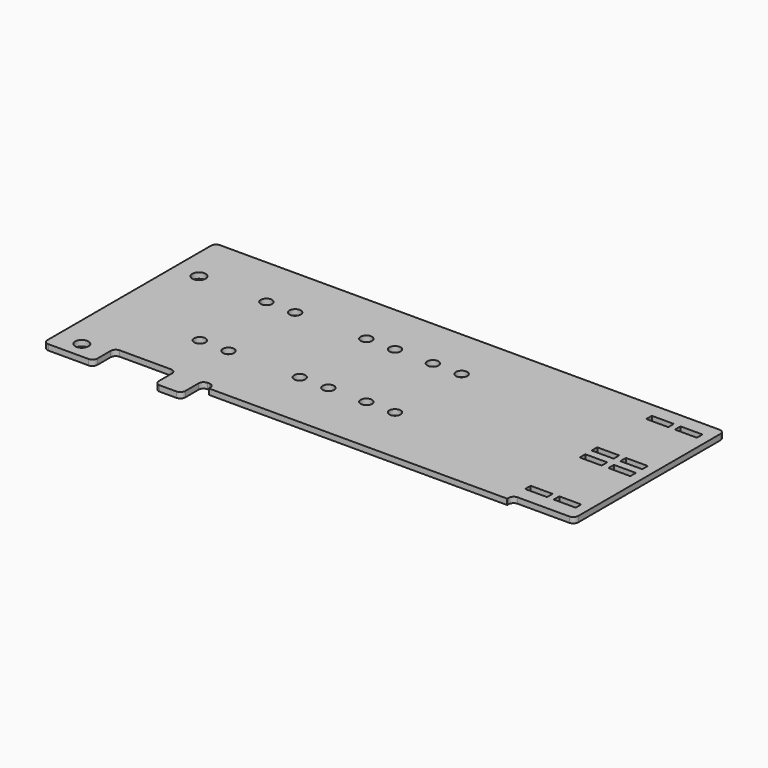
from build123d import *

# Parameters (mm, degrees)
F0_W     = 153
F0_H     = 69
F1_DEPTH = 1.7
F2_W     = 15
F2_H     = 4.6
F2_W_2   = 8
F2_W_3   = 1.9
F2_H_2   = 8.5
F2_W_4   = 18.5
F2_H_3   = 12.6
F2_R     = 2
F2_W_5   = 6.6
F2_H_4   = 2.1
F2_R_2   = 1.7
F3_DEPTH = 1.701
F4_W     = 89.6
F4_H     = 10.55
F5_DEPTH = 1.701
F6_R     = 1.5


with BuildPart() as f1:
    # F0 (on Top) → F1 (new body)
    with BuildSketch(Plane.XY):
        Rectangle(F0_W, F0_H)
    extrude(amount=F1_DEPTH)

    # F2 (on face) → F3 (cut, through all)
    with BuildSketch(Plane.XY.offset(1.7)):
        with Locations((-69, -32.2)):
            Rectangle(F2_W, F2_H)
        Polygon((-61.5, -29.9), (-61.5, -34.5), (-43.1, -34.5), (-43.1, -29.9), (-43.1, -21.9), (-61.5, -21.9), align=None)
        with Locations((-39.1, -32.2)):
            Rectangle(F2_W_2, F2_H)
        Polygon((-35.1, -29.9), (-35.1, -34.5), (-31.6, -34.5), (-31.6, -21.9), (-35.1, -21.9), align=None)
        with Locations((-19.35, -30.25)):
            Rectangle(F2_W_3, F2_H_2)
        with Locations((67.25, -28.2)):
            Rectangle(F2_W_4, F2_H_3)
        with Locations((-69, -24.9)):
            Circle(F2_R)
        with Locations((-69, 19.1)):
            Circle(F2_R)
        with Locations((61.5, 29.05)):
            Rectangle(F2_W_5, F2_H_4)
        with Locations((61.5, 8.55)):
            Rectangle(F2_W_5, F2_H_4)
        with Locations((-48.5, 18.8)):
            Circle(F2_R_2)
        with Locations((-18.5, 18.8)):
            Circle(F2_R_2)
        with Locations((1.5, 18.8)):
            Circle(F2_R_2)
        with Locations((-39.9, 18.8)):
            Circle(F2_R_2)
        with Locations((-9.9, 18.8)):
            Circle(F2_R_2)
        with Locations((10.1, 18.8)):
            Circle(F2_R_2)
        with Locations((70.1, 8.55)):
            Rectangle(F2_W_5, F2_H_4)
        with Locations((70.1, 29.05)):
            Rectangle(F2_W_5, F2_H_4)
        with Locations((70.1, -16.45)):
            Rectangle(F2_W_5, F2_H_4)
        with Locations((61.5, 4.05)):
            Rectangle(F2_W_5, F2_H_4)
        with Locations((70.1, 4.05)):
            Rectangle(F2_W_5, F2_H_4)
        with Locations((61.5, -16.45)):
            Rectangle(F2_W_5, F2_H_4)
        with Locations((1.5, -6.2)):
            Circle(F2_R_2)
        with Locations((-18.5, -6.2)):
            Circle(F2_R_2)
        with Locations((-9.9, -6.2)):
            Circle(F2_R_2)
        with Locations((10.1, -6.2)):
            Circle(F2_R_2)
        with Locations((-39.9, -6.2)):
            Circle(F2_R_2)
        with Locations((-48.5, -6.2)):
            Circle(F2_R_2)
    extrude(amount=-F3_DEPTH, mode=Mode.SUBTRACT)

    # F4 (on Top) → F5 (cut, through all)
    with BuildSketch(Plane.XY):
        with Locations((13.2, -29.225)):
            Rectangle(F4_W, F4_H)
    extrude(amount=F5_DEPTH, mode=Mode.SUBTRACT)

    # F6
    f6_edges = [f1.edges().sort_by_distance(p)[0] for p in [
        (-35.1, -21.9, 0.85),
        (-31.6, -21.9, 0.85),
        (-43.1, -21.9, 0.85),
        (58, -21.9, 0.85),
        (76.5, -21.9, 0.85),
        (-35.1, -29.9, 0.85),
        (-43.1, -29.9, 0.85),
        (-76.5, -29.9, 0.85),
        (-61.5, -29.9, 0.85),
        (-61.5, -21.9, 0.85),
        (76.5, 34.5, 0.85),
        (-76.5, 34.5, 0.85),
    ]]
    fillet(f6_edges, radius=F6_R)


solid = f1.part
